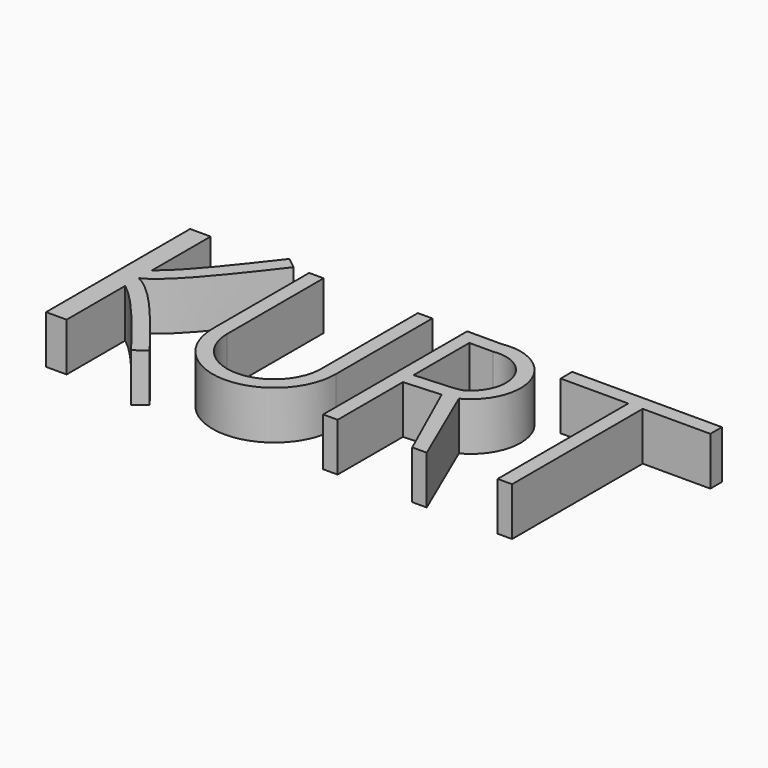
from build123d import *

# Parameters (mm, degrees)
F1_DEPTH = 25.4


# Not quite as in the source:
# - ends of sketch curves that miss each other by under 0.0002 mm in the source are joined
# - the dataset's text gives a spline's control points without its knots; the knots are read off the source's solid


with BuildPart() as f1:
    # F0 (on Top) → F1 (new body)
    with BuildSketch(Plane.XY):
        with BuildLine():
            Line((-84.7116485238, 40.7445728779), (-95.5141410232, 40.7445728779))
            Line((-95.5141410232, 40.7445728779), (-95.5141410232, -6.6390763968))
            add(Edge.make_bspline(
                [(-95.5141410232, -6.6390763968), (-92.2564229583, -5.7000227681), (-88.9987048935, -4.7609691395), (-84.7116485238, -6.6390763968)],
                knots=[0, 0, 0, 0, 0.2904648184, 0.2904648184, 0.2904648184, 0.2904648184], degree=3))
            Line((-84.7116485238, -6.6390763968), (-84.7116485238, 2.2007589152))
            Line((-84.7116485238, 2.2007589152), (-84.7116485238, 40.7445728779))
        make_face()
        with BuildLine():
            add(Edge.make_bspline(
                [(-95.5141410232, -6.6390763968), (-92.2564229583, -7.5781300255), (-88.9987048935, -8.5171836542), (-84.7116485238, -6.6390763968)],
                knots=[0, 0, 0, 0, 0.2904648184, 0.2904648184, 0.2904648184, 0.2904648184], degree=3))
            Line((-95.5141410232, -6.6390763968), (-95.5141410232, -54.0227256715))
            Line((-95.5141410232, -54.0227256715), (-84.7116485238, -54.0227256715))
            Line((-84.7116485238, -54.0227256715), (-84.7116485238, -15.4789117092))
            Line((-84.7116485238, -15.4789117092), (-84.7116485238, -6.6390763968))
        make_face()
        with BuildLine():
            add(Edge.make_bspline(
                [(-95.5141410232, -6.6390763968), (-92.2564229583, -5.7000227681), (-88.9987048935, -4.7609691395), (-84.7116485238, -6.6390763968)],
                knots=[0, 0, 0, 0, 0.2904648184, 0.2904648184, 0.2904648184, 0.2904648184], degree=3))
            add(Edge.make_bspline(
                [(-95.5141410232, -6.6390763968), (-92.2564229583, -7.5781300255), (-88.9987048935, -8.5171836542), (-84.7116485238, -6.6390763968)],
                knots=[0, 0, 0, 0, 0.2904648184, 0.2904648184, 0.2904648184, 0.2904648184], degree=3))
        make_face()
        with BuildLine():
            add(Edge.make_bspline(
                [(-84.7117154486, 2.2007589152), (-83.9995557093, 2.721358536), (-82.2984407254, 4.0678338376), (-79.3197247041, 6.7769854886), (-75.8651516776, 10.2660987459), (-72.166048126, 14.2950229097), (-68.2697421496, 18.7810126405), (-62.8627961927, 25.267445643), (-55.7912554843, 34.1333862174), (-49.9563950251, 41.6480964378), (-47.0294138372, 45.4178080531)],
                knots=[0.3849384709, 0.3849384709, 0.3849384709, 0.3849384709, 0.4375, 0.5, 0.5625, 0.625, 0.6875, 0.75, 0.875, 1, 1, 1, 1], degree=3))
            Line((-84.7117154486, 2.2007589152), (-84.7116485238, -6.6390763968))
            add(Edge.make_bspline(
                [(-84.7116485238, -6.6390763968), (-74.2394084221, -2.0513153692), (-57.625039393, 19.3466287543), (-41.0106703639, 40.7445728779)],
                knots=[0.2904648184, 0.2904648184, 0.2904648184, 0.2904648184, 1, 1, 1, 1], degree=3))
            Line((-41.0106703639, 40.7445728779), (-47.0294138372, 45.4178080531))
        make_face()
        with BuildLine():
            add(Edge.make_bspline(
                [(-84.7116485238, -6.6390763968), (-74.2394084221, -11.2268374245), (-57.625039393, -32.624781548), (-41.0106703639, -54.0227256715)],
                knots=[0.2904648184, 0.2904648184, 0.2904648184, 0.2904648184, 1, 1, 1, 1], degree=3))
            Line((-84.7116485238, -6.6390763968), (-84.7116485238, -15.4789117092))
            add(Edge.make_bspline(
                [(-84.7116485238, -15.4789117092), (-83.999555709, -15.9995113299), (-82.2984407252, -17.3459866313), (-79.3197247041, -20.0551382822), (-75.8651516776, -23.5442515395), (-72.166048126, -27.5731757034), (-68.2697421496, -32.0591654341), (-62.8627961927, -38.5455984366), (-55.7912554843, -47.411539011), (-49.9563950251, -54.9262492315), (-47.0294138372, -58.6959608468)],
                knots=[0.3849384709, 0.3849384709, 0.3849384709, 0.3849384709, 0.4375, 0.5, 0.5625, 0.625, 0.6875, 0.75, 0.875, 1, 1, 1, 1], degree=3))
            Line((-47.0294138372, -58.6959608468), (-41.0106703639, -54.0227256715))
        make_face()
    extrude(amount=F1_DEPTH)


with BuildPart() as f1b:
    # F0 (on Top) → F1, piece 2 (new body)
    with BuildSketch(Plane.XY):
        with BuildLine():
            Line((-25.2555142003, -22.7554271221), (-25.2555142003, 40.7445728779))
            Line((-25.2555142003, 40.7445728779), (-32.8755142003, 40.7445728779))
            Line((-32.8755142003, 40.7445728779), (-32.8755142003, -22.7554271221))
            ThreePointArc((-32.8755142003, -22.7554271221), (-0.458891395, -55.1720499274), (31.9577314103, -22.7554271221))
            Line((31.9577314103, -22.7554271221), (31.9577314103, 40.7445728779))
            Line((31.9577314103, 40.7445728779), (24.3377314103, 40.7445728779))
            Line((24.3377314103, 40.7445728779), (24.3377314103, -22.7554271221))
            ThreePointArc((24.3377314103, -22.7554271221), (-0.458891395, -47.5520499274), (-25.2555142003, -22.7554271221))
        make_face()
    extrude(amount=F1_DEPTH)


with BuildPart() as f1c:
    # F0 (on Top) → F1, piece 3 (new body)
    with BuildSketch(Plane.XY):
        with BuildLine():
            Line((68.4872940183, 40.7445728779), (50.3194704652, 40.7445728779))
            Line((50.3194704652, 40.7445728779), (50.3194704652, -54.0227256715))
            Line((50.3194704652, -54.0227256715), (57.9303130507, -54.0227256715))
            Line((57.9303130507, -54.0227256715), (57.9303130507, -11.0582793131))
            Line((57.9303130507, -11.0582793131), (77.325694263, -9.8307235166))
            Line((77.325694263, -9.8307235166), (97.2029411244, -54.0227256715))
            Line((97.2029411244, -54.0227256715), (104.8229411244, -54.0227256715))
            Line((104.8229411244, -54.0227256715), (85.059591811, -8.1937922423))
            ThreePointArc((85.059591811, -8.1937922423), (97.6793396869, 23.3548819617), (68.4872940183, 40.7445728779))
        make_face()
        with BuildLine():
            Line((57.4489976161, 33.2341308831), (69.7747958795, 33.2341308831))
            ThreePointArc((69.7747958795, 33.2341308831), (90.4619367109, 20.9108086643), (81.5188669265, -1.4463729362))
            Line((81.5188669265, -1.4463729362), (76.8443788283, -2.225939795))
            Line((76.8443788283, -2.225939795), (57.4489976161, -3.4534955915))
            Line((57.4489976161, -3.4534955915), (57.4489976161, 33.2341308831))
        make_face(mode=Mode.SUBTRACT)
    extrude(amount=F1_DEPTH)


with BuildPart() as f1d:
    # F0 (on Top) → F1, piece 4 (new body)
    with BuildSketch(Plane.XY):
        Polygon((185.3505820036, 39.5261689079), (106.5415218472, 39.5261689079), (106.5415218472, 31.9061689079), (142.1360519254, 31.9061689079), (145.9460519254, 31.9061689079), (149.7560519254, 31.9061689079), (185.3505820036, 31.9061689079), align=None)
        Polygon((145.9460519254, 31.9061689079), (142.1360519254, 31.9061689079), (142.1360519254, -54.0227256715), (145.9460519254, -54.0227256715), (149.7560519254, -54.0227256715), (149.7560519254, 31.9061689079), align=None)
    extrude(amount=F1_DEPTH)


solid = Compound([f1.part, f1b.part, f1c.part, f1d.part])
